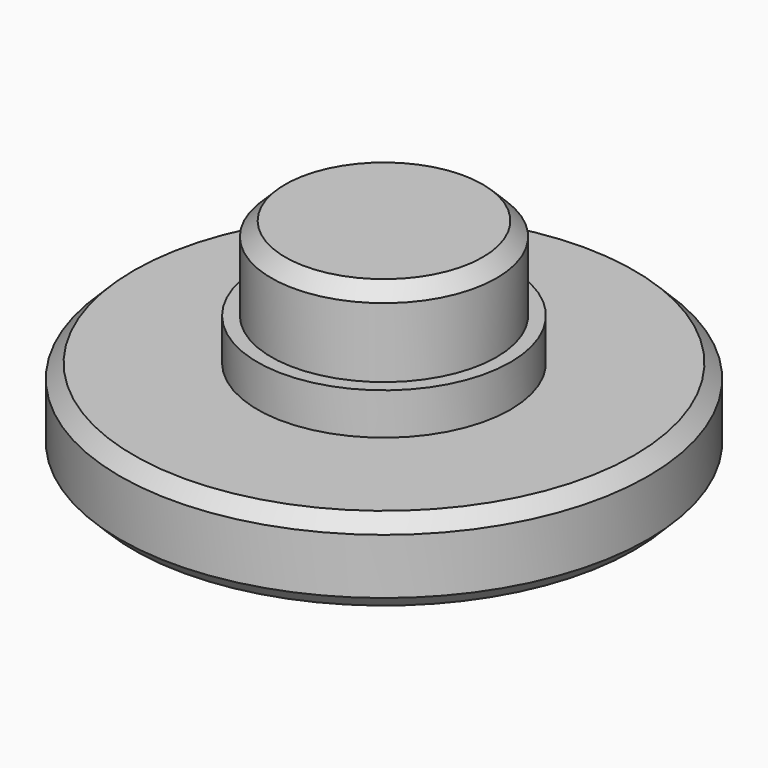
from build123d import *

# Parameters (mm, degrees)
F0_R         = 9.5
F1_DEPTH     = 3
F2_R         = 4.05
F3_DEPTH     = 4.5
F4_SIZE      = 0.5
F5_R         = 4.55
F6_DEPTH     = 1.5
F7_TEXT_SIZE = 13.8888888889
F8_DEPTH     = 1


# Not quite as in the source:
# - Text() gives the source's letters only with a copy of the font that has no kerning and outlines rounded to 1/6400 em; it was checked with that copy


with BuildPart() as f1:
    # F0 (on Top) → F1 (new body)
    with BuildSketch(Plane.XY):
        Circle(F0_R)
    extrude(amount=F1_DEPTH)

    # F2 (on face) → F3 (join)
    with BuildSketch(Plane.XY.offset(3)):
        Circle(F2_R)
    extrude(amount=F3_DEPTH)

    # F4
    f4_edges = [f1.edges().sort_by_distance(p)[0] for p in [
        (-4.05, 0, 7.5),
        (-9.5, 0, 3),
        (-9.5, 0, 0),
    ]]
    chamfer(f4_edges, length=F4_SIZE)

    # F5 (on face) → F6 (join)
    with BuildSketch(Plane.XY.offset(3)):
        Circle(F5_R)
    extrude(amount=F6_DEPTH)

    # F7 (on face) → F8 (cut)
    with BuildSketch(Plane(origin=(0, 0, 0), x_dir=(1, 0, 0), z_dir=(0, 0, -1))):
        with Locations((-5.205078125, -5)):
            Text('D', F7_TEXT_SIZE, font='Arimo', font_style=FontStyle.BOLD, text_align=(TextAlign.LEFT, TextAlign.BOTTOM))
    extrude(amount=-F8_DEPTH, mode=Mode.SUBTRACT)


solid = f1.part
